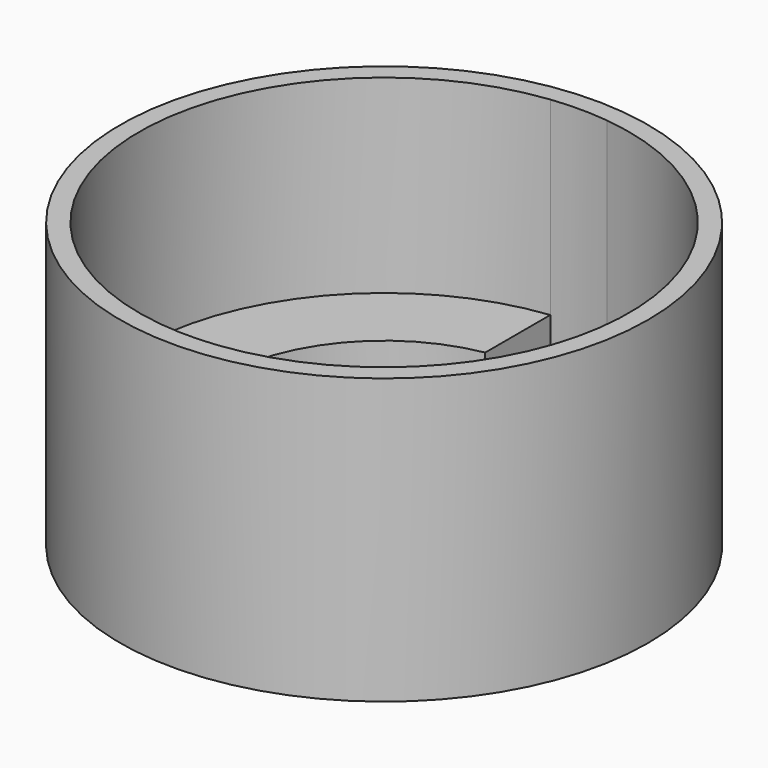
from build123d import *

# Parameters (mm, degrees)
F0_R      = 16.7
F0_R_2    = 15.5
F1_DEPTH  = 15
F2_R      = 15.5
F3_DEPTH  = 3
F4_R      = 10.4
F5_DEPTH  = 25
F6_R      = 16.7
F6_R_2    = 13.7
F7_DEPTH  = 3
F10_DEPTH = 25


# Not quite as in the source:
# - a pattern or mirror of a feature is missing from the dataset's text; its kind, count and spacing are read off the source's solid


with BuildPart() as f1:
    # F0 (on Top) → F1 (new body)
    with BuildSketch(Plane.XY):
        Circle(F0_R)
        Circle(F0_R_2, mode=Mode.SUBTRACT)
    extrude(amount=F1_DEPTH)

    # F2 (on face) → F3 (join)
    with BuildSketch(Plane(origin=(0, 0, 0), x_dir=(1, 0, 0), z_dir=(0, 0, -1))):
        Circle(F2_R)
    extrude(amount=-F3_DEPTH)

    # F4 (on face) → F5 (cut)
    with BuildSketch(Plane.XY.offset(3)):
        Circle(F4_R)
    extrude(amount=-F5_DEPTH, mode=Mode.SUBTRACT)

    # F6 (on face) → F7 (join)
    with BuildSketch(Plane(origin=(0, 0, 0), x_dir=(1, 0, 0), z_dir=(0, 0, -1))):
        Circle(F6_R)
        Circle(F6_R_2, mode=Mode.SUBTRACT)
    extrude(amount=F7_DEPTH)

    # F9 (on face) → F10 (cut)
    with BuildSketch(Plane(origin=(0, 0, -3), x_dir=(1, 0, 0), z_dir=(0, 0, -1))):
        with BuildLine():
            Line((-1.8, 8.9434019272), (1.8, 8.9434019272))
            Line((1.8, 8.9434019272), (1.8, 13.5812370571))
            ThreePointArc((1.8, 13.5812370571), (0, 13.7), (-1.8, 13.5812370571))
            Line((-1.8, 13.5812370571), (-1.8, 8.9434019272))
        make_face()
        with BuildLine():
            ThreePointArc((-1.8, 13.5812370571), (0, 13.7), (1.8, 13.5812370571))
            Line((1.8, 13.5812370571), (1.8, 15.3951290998))
            ThreePointArc((1.8, 15.3951290998), (0, 15.5), (-1.8, 15.3951290998))
            Line((-1.8, 15.3951290998), (-1.8, 13.5812370571))
        make_face()
    f10 = extrude(amount=-F10_DEPTH, mode=Mode.SUBTRACT)

    # F10_copies: F10 across plane
    add(f10.mirror(Plane.ZX), mode=Mode.SUBTRACT)


solid = f1.part
